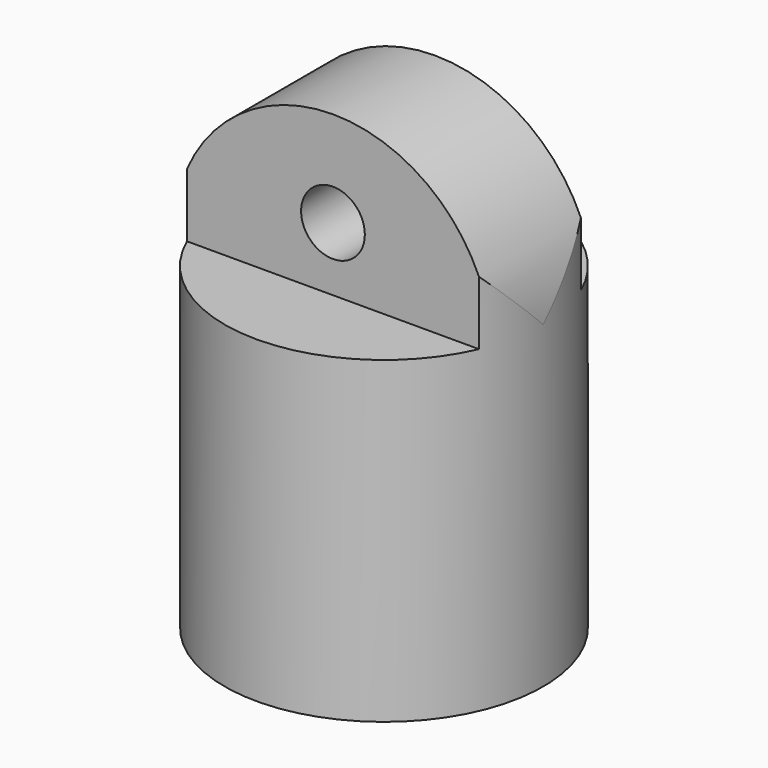
from build123d import *

# Parameters (mm, degrees)
F0_R          = 15.875
F1_DEPTH      = 31.75
F2_R          = 12.7
F3_DEPTH      = 25.4
F4_R          = 3.175
F5_DEPTH      = 6.35
F5_DEPTH_BACK = 6.35
F6_W          = 11.146276543
F6_H          = 50.8


# Not quite as in the source:
# - after a boolean that leaves OpenCascade's solid faulty, fix() repairs it


with BuildPart() as f1:
    # F0 (on Top) → F1 (new body)
    with BuildSketch(Plane.XY):
        Circle(F0_R)
    extrude(amount=F1_DEPTH)

    # F2 (on face) → F3 (cut)
    with BuildSketch(Plane(origin=(0, 0, 0), x_dir=(1, 0, 0), z_dir=(0, 0, -1))):
        Circle(F2_R)
    extrude(amount=-F3_DEPTH, mode=Mode.SUBTRACT)

    # F4 (on Front) → F5 (join, two sides)
    with BuildSketch(Plane.XZ) as f5_sk:
        with BuildLine():
            ThreePointArc((15.875, 31.75), (0, 47.625), (-15.875, 31.75))
            Line((-15.875, 31.75), (15.875, 31.75))
        make_face()
        with Locations((0, 38.1)):
            Circle(F4_R, mode=Mode.SUBTRACT)
    extrude(amount=F5_DEPTH)
    extrude(f5_sk.sketch, amount=-F5_DEPTH_BACK)

    # F6 (on Front) → F7 (revolve, cut)
    with BuildSketch(Plane.XZ):
        with Locations((-21.4481382715, 25.4)):
            Rectangle(F6_W, F6_H)
    revolve(axis=Axis((0, 0, 12.5730000436), (0, 0, 1)), mode=Mode.SUBTRACT)

    add(f1.part.fix(), mode=Mode.REPLACE)


solid = f1.part
